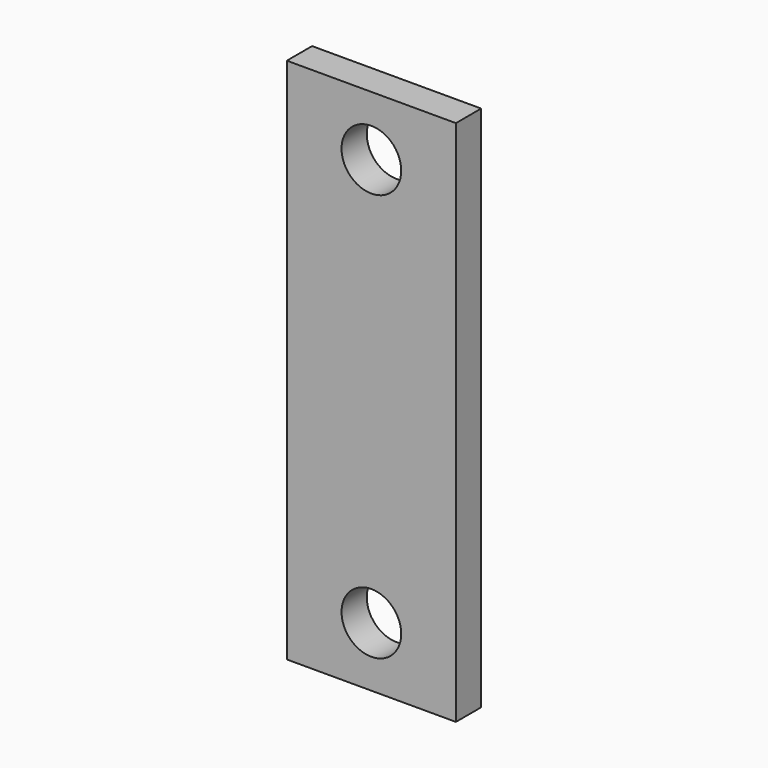
from build123d import *

# Parameters (mm, degrees)
F0_W     = 17
F0_H     = 53
F0_R     = 3
F1_DEPTH = 3.175


# Not quite as in the source:
# - a length typed as a fraction of an inch, garbled in the dataset ("3 / 203.2 mm" for 3/8 in), is restored


with BuildPart() as f1:
    # F0 (on Front) → F1 (new body)
    with BuildSketch(Plane.XZ):
        Rectangle(F0_W, F0_H)
        with Locations((0, -20.5)):
            Circle(F0_R, mode=Mode.SUBTRACT)
        with Locations((0, 20.5)):
            Circle(F0_R, mode=Mode.SUBTRACT)
    extrude(amount=F1_DEPTH)


solid = f1.part
